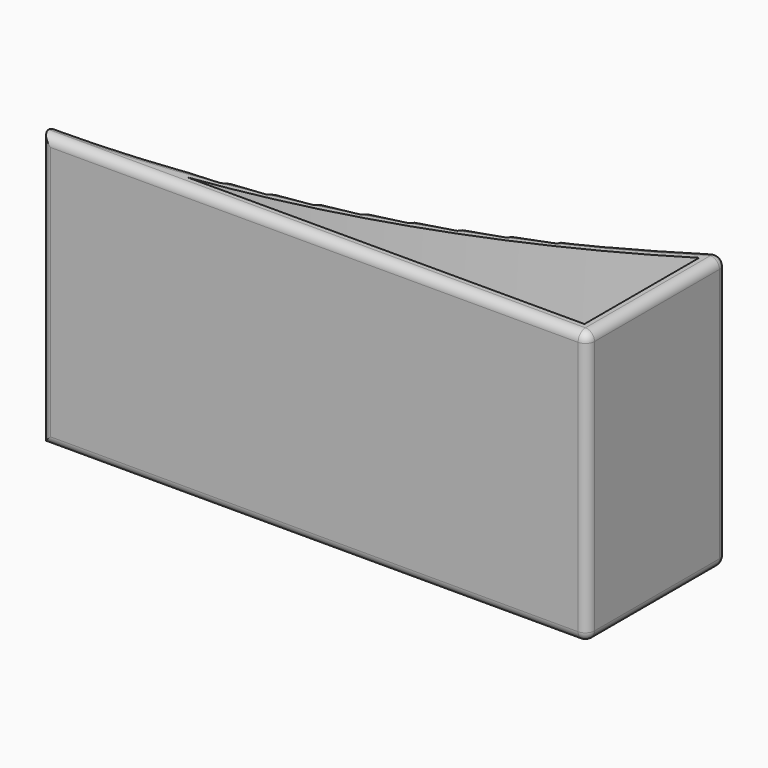
from build123d import *

# Parameters (mm, degrees)
F1_DEPTH = 30
F2_T     = -1.5
F3_R     = 0.99999


# Not quite as in the source:
# - a fillet or chamfer is up to 0.001 mm smaller than in the source, because OpenCascade refuses the exact size


with BuildPart() as f1:
    # F0 (on Top) → F1 (new body)
    with BuildSketch(Plane.XY):
        with BuildLine():
            Line((-60, 2), (-60, 0))
            Line((-60, 0), (0, 0))
            Line((0, 0), (0, 20))
            ThreePointArc((0, 20), (-28.6790804733, 6.5969349109), (-60, 2))
        make_face()
    extrude(amount=F1_DEPTH)

    # F2
    f2_openings = [f1.faces().sort_by_distance(p)[0] for p in [
        (-18.660264, 5.692192, 30),
        (-18.660264, 5.692192, 0),
    ]]
    offset(amount=F2_T, openings=f2_openings)

    # F3 (radius 1 in the source; OpenCascade refuses exactly that, so slightly less here)
    f3_edges = [f1.edges().sort_by_distance(p)[0] for p in [
        (-60, 2, 15),
        (-60, 0, 15),
        (-28.67908, 6.596935, 30),
        (-30, 0, 30),
        (-28.67908, 6.596935, 0),
        (-30, 0, 0),
        (0, 20, 15),
        (0, 0, 15),
        (0, 10, 30),
        (0, 10, 0),
    ]]
    fillet(f3_edges, radius=F3_R)


solid = f1.part
